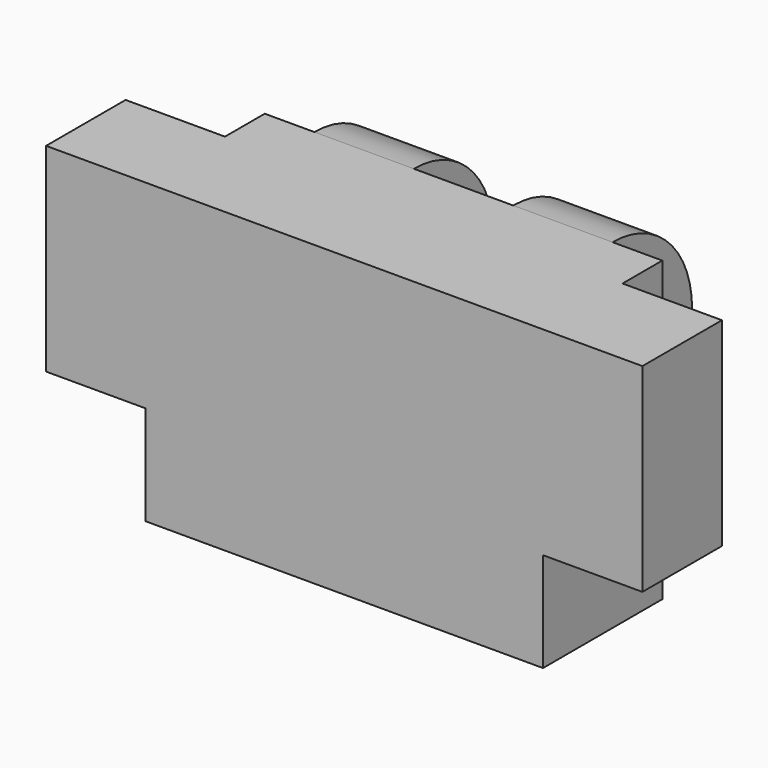
from build123d import *

# Parameters (mm, degrees)
F0_W     = 100
F0_H     = 12.5
F1_DEPTH = 50
F2_W     = 25
F2_H     = 50
F3_DEPTH = 25
F4_R     = 24.99999
F5_R     = 5
F6_DEPTH = 112.501
F7_W     = 50
F7_H     = 10
F8_DEPTH = 75


# Not quite as in the source:
# - a fillet or chamfer is up to 0.001 mm smaller than in the source, because OpenCascade refuses the exact size


with BuildPart() as f1:
    # F0 (on Top) → F1 (new body)
    with BuildSketch(Plane.XY):
        Polygon((75, -12.5), (75, 12.5), (50, 12.5), (50, 0), (-50, 0), (-50, 12.5), (-75, 12.5), (-75, -12.5), align=None)
        with Locations((0, 6.25)):
            Rectangle(F0_W, F0_H)
        with Locations((0, 18.75)):
            Rectangle(F0_W, F0_H)
    extrude(amount=F1_DEPTH)

    # F2 (on face) → F3 (join)
    with BuildSketch(Plane(origin=(0, 25, 0), x_dir=(-1, 0, 0), z_dir=(0, 1, 0))):
        with Locations((-25, 25)):
            Rectangle(F2_W, F2_H)
        with Locations((25, 25)):
            Rectangle(F2_W, F2_H)
    extrude(amount=F3_DEPTH)

    # F4 (radius 25 in the source; OpenCascade refuses exactly that, so slightly less here)
    f4_edges = [f1.edges().sort_by_distance(p)[0] for p in [
        (25, 50, 50),
        (25, 50, 0),
        (-25, 50, 0),
        (-25, 50, 50),
    ]]
    fillet(f4_edges, radius=F4_R)

    # F5 (on face) → F6 (cut, through all)
    with BuildSketch(Plane.YZ.offset(37.5)):
        with Locations((38.875002414, 25)):
            Circle(F5_R)
    extrude(amount=-F6_DEPTH, mode=Mode.SUBTRACT)

    # F7 (on face) → F8 (join)
    with BuildSketch(Plane.XY.offset(50)):
        Polygon((25, 25), (25, -2.5), (25, -12.5), (50, -12.5), (50, 12.5), (50, 25), (37.5, 25), align=None)
        with Locations((0, -7.5)):
            Rectangle(F7_W, F7_H)
        Polygon((-37.5, 25), (-50, 25), (-50, 12.5), (-50, -12.5), (-25, -12.5), (-25, -2.5), (-25, 25), align=None)
    extrude(amount=-F8_DEPTH)


solid = f1.part
